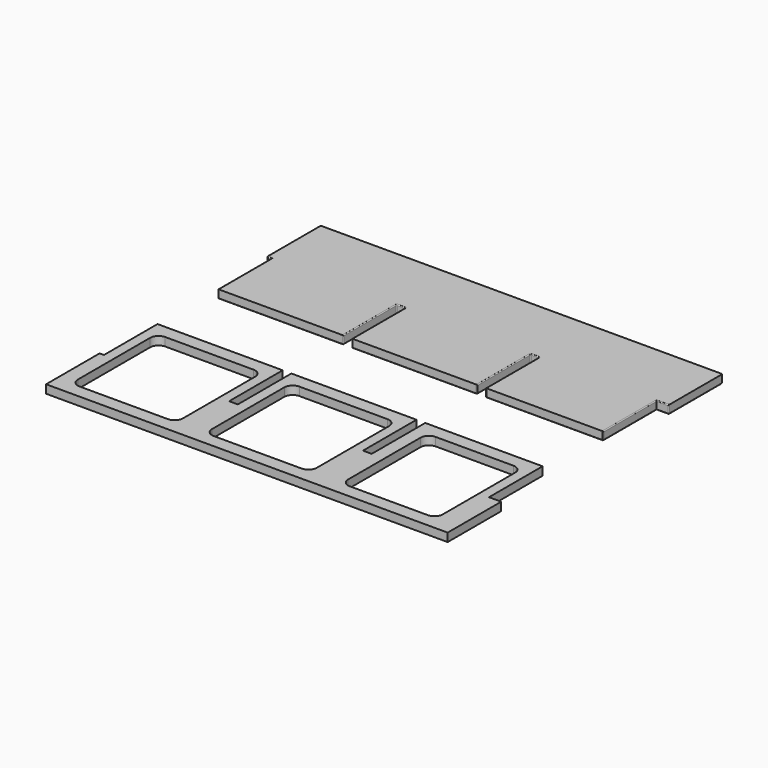
from build123d import *

# Parameters (mm, degrees)
F1_DEPTH = 5
F0_W     = 62.8
F0_H     = 64
F0_W_2   = 62.635196808
F0_W_3   = 56.5503612161
F2_R     = 0.5
F3_R     = 5


with BuildPart() as f1:
    # F0 (on Top) → F1 (new body)
    with BuildSketch(Plane.XY):
        Polygon((120, 40), (-120, 40), (-120, 0), (-117.4, 0), (-117.4, -40), (-42.6, -40), (-42.6, 0), (-37.4, 0), (-37.4, -40), (37.4, -40), (37.4, 0), (42.6, 0), (42.6, -40), (112.7228473783, -40), (112.7228473783, 0), (120, 0), align=None)
    extrude(amount=F1_DEPTH)

    # F2
    f2_edges = [f1.edges().sort_by_distance(p)[0] for p in [
        (-42.6, -40, 2.5),
        (-37.4, -40, 2.5),
        (37.4, -40, 2.5),
        (42.6, -40, 2.5),
        (-120, 40, 2.5),
        (120, 40, 2.5),
        (42.6, 0, 2.5),
        (37.4, 0, 2.5),
        (-37.4, 0, 2.5),
        (-42.6, 0, 2.5),
        (-40, 0, 0),
        (0, 40, 0),
        (-120, 20, 0),
        (-118.7, 0, 0),
        (-117.4, -20, 0),
        (-80, -40, 0),
        (-42.6, -20, 0),
        (-37.4, -20, 0),
        (0, -40, 0),
        (37.4, -20, 0),
        (40, 0, 0),
        (42.6, -20, 0),
        (77.661424, -40, 0),
        (112.722847, -20, 0),
        (116.361424, 0, 0),
        (120, 20, 0),
        (-40, 0, 5),
        (40, 0, 5),
        (-117.4, -20, 5),
        (-118.7, 0, 5),
        (112.722847, -20, 5),
        (116.361424, 0, 5),
        (-120, 0, 2.5),
        (-117.4, -40, 2.5),
        (-42.6, -20, 5),
        (-37.4, -20, 5),
        (37.4, -20, 5),
        (42.6, -20, 5),
        (112.722847, -40, 2.5),
        (120, 0, 2.5),
    ]]
    fillet(f2_edges, radius=F2_R)


with BuildPart() as f1b:
    # F0 (on Top) → F1, piece 2 (new body)
    with BuildSketch(Plane.XY):
        Polygon((-42.6, -85.212714076), (-117.4, -85.212714076), (-117.4, -125.212714076), (-120, -125.212714076), (-120, -165.212714076), (120, -165.212714076), (120, -125.212714076), (112.7228473783, -125.212714076), (112.7228473783, -85.212714076), (42.6, -85.212714076), (42.6, -125.212714076), (37.4, -125.212714076), (37.4, -85.212714076), (-37.4, -85.212714076), (-37.4, -125.212714076), (-42.6, -125.212714076), align=None)
        with Locations((-80, -125.212714076)):
            Rectangle(F0_W, F0_H, mode=Mode.SUBTRACT)
        with Locations((0.082401596, -125.212714076)):
            Rectangle(F0_W_2, F0_H, mode=Mode.SUBTRACT)
        with Locations((78.4476667702, -125.212714076)):
            Rectangle(F0_W_3, F0_H, mode=Mode.SUBTRACT)
    extrude(amount=F1_DEPTH)

    # F3
    f3_edges = [f1b.edges().sort_by_distance(p)[0] for p in [
        (-111.4, -93.212714, 2.5),
        (-48.6, -93.212714, 2.5),
        (-111.4, -157.212714, 2.5),
        (-48.6, -157.212714, 2.5),
        (106.722847, -93.212714, 2.5),
        (31.4, -93.212714, 2.5),
        (31.4, -157.212714, 2.5),
        (106.722847, -157.212714, 2.5),
        (50.172486, -157.212714, 2.5),
        (-31.235197, -157.212714, 2.5),
        (-31.235197, -93.212714, 2.5),
        (50.172486, -93.212714, 2.5),
    ]]
    fillet(f3_edges, radius=F3_R)


solid = Compound([f1.part, f1b.part])
